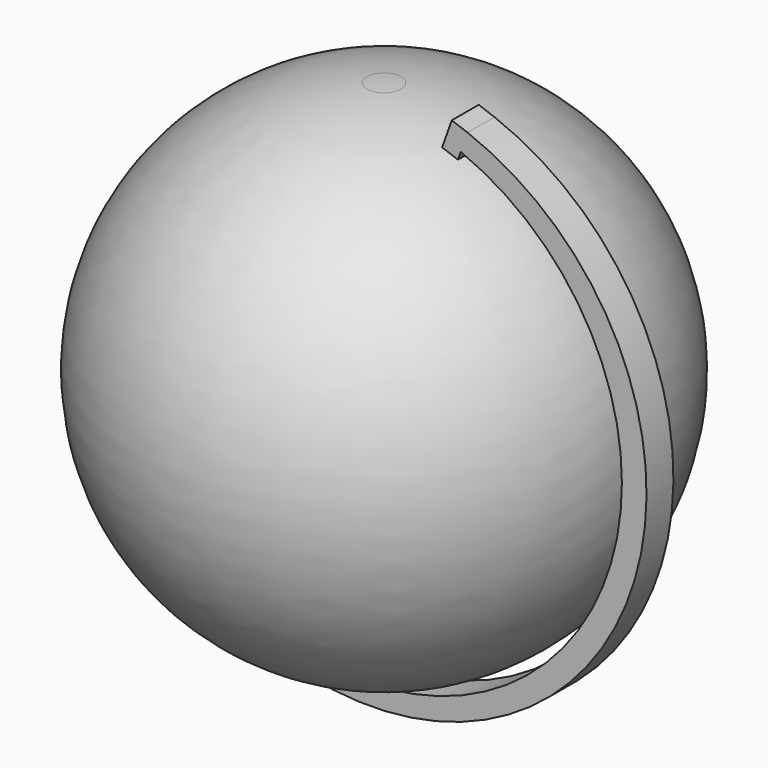
from build123d import *

# Parameters (mm, degrees)
F3_DEPTH = 10.16


# Not quite as in the source:
# - a feature of the source that left no trace in its solid (it failed there, or was rolled back) is left out


with BuildPart() as f1:
    # F0 (on Front) → F1 (revolve)
    with BuildSketch(Plane.XZ):
        with BuildLine():
            ThreePointArc((5.1168156788, 75.8314730669), (2.5598933329, 75.9629165328), (0, 76.0084729955))
            Line((0, 76.0084729955), (0, -76.545633716))
            ThreePointArc((0, -76.545633716), (76.1568791815, -2.8330299886), (5.1258229017, 75.830857779))
            Line((5.1258229017, 75.830857779), (5.1168156788, 75.8314730669))
        make_face()
    revolve(axis=Axis((0, 0, -0.2685803602), (0, 0, -1)))

    # F2 (on Front) → F3 (join)
    with BuildSketch(Plane.XZ):
        Polygon((31.3011850432, 71.831902576), (33.3672479498, 77.6121955782), (28.5836376165, 79.322011995), (25.6679828013, 71.164787415), (30.4515931346, 69.4549709982), align=None)
        with BuildLine():
            Line((-21.0232065567, -75.0018807282), (-22.6610616984, -80.2421604659))
            ThreePointArc((-22.6610616984, -80.2421604659), (82.5983967155, -28.7321782492), (33.3672479498, 77.6121955782))
            Line((33.3672479498, 77.6121955782), (31.3011850432, 71.831902576))
            ThreePointArc((31.3011850432, 71.831902576), (75.4556591104, -26.642417192), (-21.0232065567, -75.0018807282))
        make_face()
    extrude(amount=F3_DEPTH)


solid = f1.part
